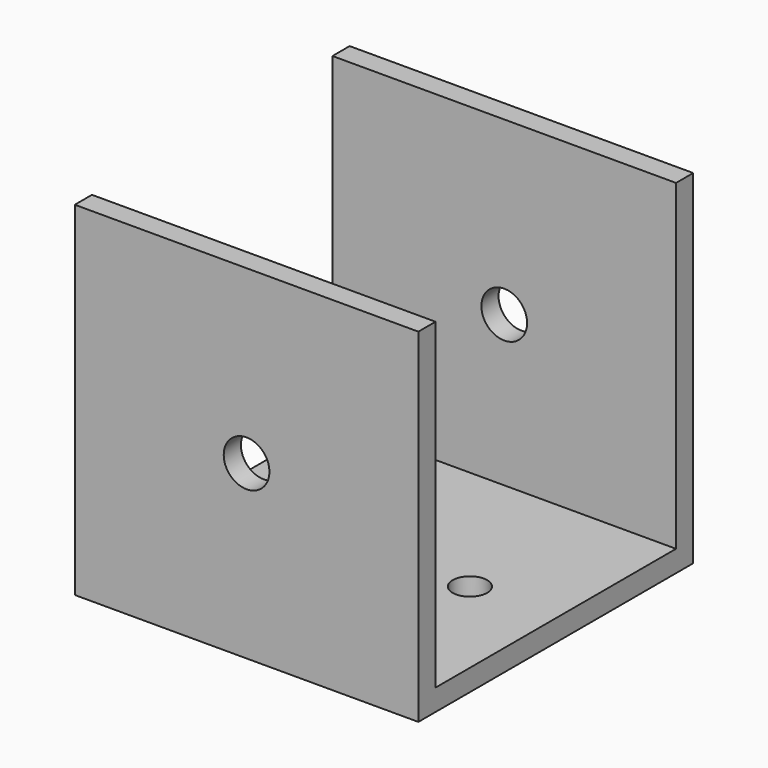
from build123d import *

# Parameters (mm, degrees)
F1_DEPTH = 25.4
F3_D     = 5.1054
F5_D     = 6.7564


with BuildPart() as f1:
    # F0 (on Right) → F1 (new body, symmetric)
    with BuildSketch(Plane.YZ):
        Polygon((-25.4, 50.8), (-25.4, 0), (0, 0), (0, 3.175), (-22.225, 3.175), (-22.225, 50.8), align=None)
        Polygon((0, 3.175), (0, 0), (25.4, 0), (25.4, 50.8), (22.225, 50.8), (22.225, 3.175), align=None)
    extrude(amount=F1_DEPTH, both=True)

    # F3 (through all)
    with Locations(Plane.XY.offset(3.175)):
        with Locations((-12.7, 0), (12.7, 0)):
            Hole(F3_D / 2)

    # F5 (through all)
    with Locations(Plane.XZ.offset(25.4)):
        with Locations((0, 25.4)):
            Hole(F5_D / 2)


solid = f1.part
